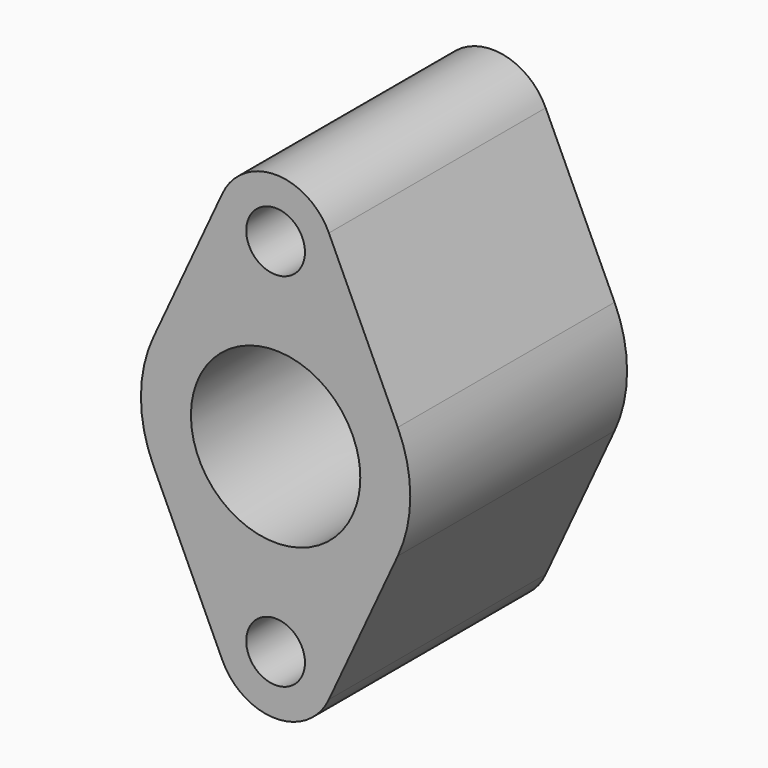
from build123d import *

# Parameters (mm, degrees)
F0_R     = 6.5
F1_DEPTH = 60
F3_ANGLE = 90


# Not quite as in the source:
# - a feature names something its author has since deleted; it is built from what else it names


with BuildPart() as f1:
    # F0 (on Front) → F1 (new body)
    with BuildSketch(Plane.XZ):
        with BuildLine():
            Line((-11.7955299893, 45.4649311314), (-27.0527510662, 12.5336819647))
            ThreePointArc((-27.0527510662, 12.5336819647), (-29.8151727119, 0), (-27.0527510662, -12.5336819647))
            Line((-27.0527510662, -12.5336819647), (-11.7955299893, -45.4649311314))
            ThreePointArc((-11.7955299893, -45.4649311314), (0, -53), (11.7955299893, -45.4649311314))
            Line((11.7955299893, -45.4649311314), (27.0527510662, -12.5336819647))
            ThreePointArc((27.0527510662, -12.5336819647), (29.8151727119, 0), (27.0527510662, 12.5336819647))
            Line((27.0527510662, 12.5336819647), (11.7955299893, 45.4649311314))
            ThreePointArc((11.7955299893, 45.4649311314), (0, 53), (-11.7955299893, 45.4649311314))
        make_face()
        with Locations((0, -40)):
            Circle(F0_R, mode=Mode.SUBTRACT)
        with BuildLine():
            ThreePointArc((17.9448621018, -5.4354782815), (-18.75, 0), (17.9448621018, 5.4354782815))
            ThreePointArc((17.9448621018, 5.4354782815), (24.1748678936, 5.401139318), (27.28, 0))
            ThreePointArc((27.28, 0), (24.1748678936, -5.401139318), (17.9448621018, -5.4354782815))
        make_face(mode=Mode.SUBTRACT)
        with Locations((0, 40)):
            Circle(F0_R, mode=Mode.SUBTRACT)
        with BuildLine():
            ThreePointArc((17.9448621018, 5.4354782815), (18.5476233573, 2.7473929089), (18.75, 0))
            ThreePointArc((18.75, 0), (18.5476233573, -2.7473929089), (17.9448621018, -5.4354782815))
            ThreePointArc((17.9448621018, -5.4354782815), (24.1748678936, -5.401139318), (27.28, 0))
            ThreePointArc((27.28, 0), (24.1748678936, 5.401139318), (17.9448621018, 5.4354782815))
        make_face()
    extrude(amount=F1_DEPTH)


with BuildPart() as f2:
    # F0 (on Front) → F2 (revolve)
    with BuildSketch(Plane.XZ):
        with BuildLine():
            ThreePointArc((78.6849431597, 21.03), (68.9626292834, 15.8333148696), (70.0431715295, 26.8042470045))
            Line((70.0431715295, 26.8042470045), (65.4349431597, 24.8954563152))
            Line((65.4349431597, 24.8954563152), (65.4349431597, 0))
            Line((65.4349431597, 0), (79.4349431597, 0))
            Line((79.4349431597, 0), (79.4349431597, 24.8954563152))
            Line((79.4349431597, 24.8954563152), (74.8267146878, 26.8042470468))
            ThreePointArc((74.8267146878, 26.8042470468), (77.6316282594, 24.5023139222), (78.6849431597, 21.03))
        make_face()
        with BuildLine():
            ThreePointArc((74.8267146878, 26.8042470468), (72.4349431044, 27.28), (70.0431715295, 26.8042470045))
            ThreePointArc((70.0431715295, 26.8042470045), (68.9626292834, 15.8333148696), (78.6849431597, 21.03))
            ThreePointArc((78.6849431597, 21.03), (77.6316282594, 24.5023139222), (74.8267146878, 26.8042470468))
        make_face()
    revolve(axis=Axis((72.4349431597, 0, 0), (1, 0, 0)))


with BuildPart() as f2_1:
    # F3: moved
    add(f2.part.rotate(Axis((72.4349431597, 0, 17.3734594136), (0, 0, 1)), F3_ANGLE))


with BuildPart() as f2_2:
    # F4: moved
    add(f2_1.part.moved(Location((-72.7008, -12.31385, -0.07673))))


with BuildPart() as f1_1:
    add(f1.part)

    # F5: cut F2
    add(f2_2.part, mode=Mode.SUBTRACT)


solid = f1_1.part
